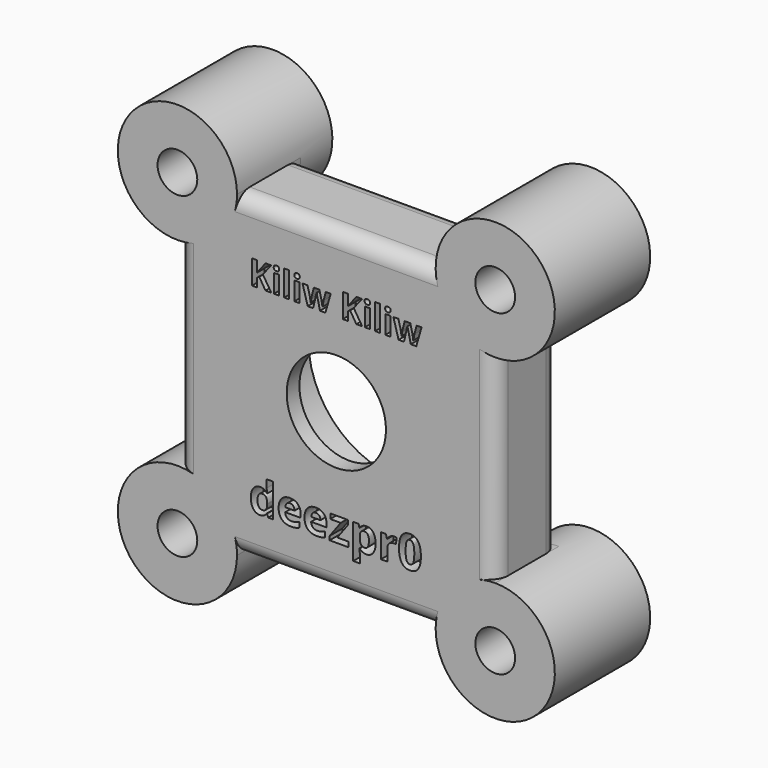
from build123d import *

# Parameters (mm, degrees)
F0_W            = 40
F0_H            = 40
F1_DEPTH        = 5
F2_R            = 11.5
F3_DEPTH        = 8
F4_R            = 6.25
F5_DEPTH        = 25
F7_DEPTH        = 15
F8_R            = 2.5
F9_DEPTH        = 35
F10_T4_DEPTH    = 35
F10_S5_R        = 7.5
F10_T6_DEPTH    = 19
F10_S7_R        = 7.5
F10_T8_DEPTH    = 19
F10_T12_DEPTH   = 35
F10_S13_R       = 7.5
F10_T14_DEPTH   = 19
F10_S15_R       = 7.5
F10_T16_DEPTH   = 19
F10_T20_DEPTH   = 35
F10_S21_R       = 7.5
F10_T22_DEPTH   = 19
F10_S23_R       = 7.5
F10_T24_DEPTH   = 19
F10_T28_DEPTH   = 35
F10_S29_R       = 7.5
F10_T30_DEPTH   = 19
F10_S31_R       = 7.5
F10_T32_DEPTH   = 19
F10_T36_DEPTH   = 35
F10_S37_R       = 7.5
F10_T38_DEPTH   = 19
F10_S39_R       = 7.5
F10_T40_DEPTH   = 19
F10_T44_DEPTH   = 35
F10_S45_R       = 7.5
F10_T46_DEPTH   = 19
F10_S47_R       = 7.5
F10_T48_DEPTH   = 19
F10_T52_DEPTH   = 35
F10_S53_R       = 7.5
F10_T54_DEPTH   = 19
F10_S55_R       = 7.5
F10_T56_DEPTH   = 19
F10_T60_DEPTH   = 35
F10_S61_R       = 7.5
F10_T62_DEPTH   = 19
F10_S63_R       = 7.5
F10_T64_DEPTH   = 19
F11_TEXT_SIZE   = 5.5150802977
F11_TEXT_SIZE_2 = 4.242241639
F12_DEPTH       = 2


# Not quite as in the source:
# - a fillet or chamfer that OpenCascade refuses, or shapes differently, is made with other operations: its cross-section is extruded or revolved along the edge and cut away or added
# - Text() gives the source's letters only with a copy of the font that has no kerning and outlines rounded to 1/6400 em; it was checked with that copy


with BuildPart() as f1:
    # F0 (on Front) → F1 (new body, symmetric)
    with BuildSketch(Plane.XZ):
        Rectangle(F0_W, F0_H)
    extrude(amount=F1_DEPTH, both=True)

    # F2 (on face) → F3 (cut)
    with BuildSketch(Plane(origin=(0, 5, 0), x_dir=(-1, 0, 0), z_dir=(0, 1, 0))):
        Circle(F2_R)
    extrude(amount=-F3_DEPTH, mode=Mode.SUBTRACT)

    # F4 (on face) → F5 (cut)
    with BuildSketch(Plane.XZ.offset(5)):
        Circle(F4_R)
    extrude(amount=-F5_DEPTH, mode=Mode.SUBTRACT)

    # F6 (on face) → F7 (join)
    with BuildSketch(Plane.XZ.offset(5)):
        with BuildLine():
            Line((-20, 20), (-12.5, 20))
            ThreePointArc((-12.5, 20), (-25.3033008589, 25.3033008589), (-20, 12.5))
            Line((-20, 12.5), (-20, 20))
        make_face()
        with BuildLine():
            ThreePointArc((-20, 12.5), (-14.6966991411, 14.6966991411), (-12.5, 20))
            Line((-12.5, 20), (-20, 20))
            Line((-20, 20), (-20, 12.5))
        make_face()
        with BuildLine():
            Line((20, 20), (12.5, 20))
            ThreePointArc((12.5, 20), (14.6966991411, 14.6966991411), (20, 12.5))
            Line((20, 12.5), (20, 20))
        make_face()
        with BuildLine():
            ThreePointArc((27.5, 20), (20, 27.5), (12.5, 20))
            Line((12.5, 20), (20, 20))
            Line((20, 20), (20, 12.5))
            ThreePointArc((20, 12.5), (25.3033008589, 14.6966991411), (27.5, 20))
        make_face()
        with BuildLine():
            ThreePointArc((-12.5, -20), (-14.6966991411, -14.6966991411), (-20, -12.5))
            Line((-20, -12.5), (-20, -20))
            Line((-20, -20), (-12.5, -20))
        make_face()
        with BuildLine():
            Line((-20, -20), (-20, -12.5))
            ThreePointArc((-20, -12.5), (-25.3033008589, -25.3033008589), (-12.5, -20))
            Line((-12.5, -20), (-20, -20))
        make_face()
        with BuildLine():
            Line((20, -20), (20, -12.5))
            ThreePointArc((20, -12.5), (14.6966991411, -14.6966991411), (12.5, -20))
            Line((12.5, -20), (20, -20))
        make_face()
        with BuildLine():
            ThreePointArc((27.5, -20), (25.3033008589, -14.6966991411), (20, -12.5))
            Line((20, -12.5), (20, -20))
            Line((20, -20), (12.5, -20))
            ThreePointArc((12.5, -20), (20, -27.5), (27.5, -20))
        make_face()
    extrude(amount=-F7_DEPTH)

    # F8 (on face) → F9 (cut)
    with BuildSketch(Plane.XZ.offset(5)):
        with Locations((-20, 20)):
            Circle(F8_R)
        with Locations((20, 20)):
            Circle(F8_R)
        with Locations((-20, -20)):
            Circle(F8_R)
        with Locations((20, -20)):
            Circle(F8_R)
    extrude(amount=-F9_DEPTH, mode=Mode.SUBTRACT)

    # F10: fillet of radius 2 on 8 edges, made by hand


with BuildPart() as f10_tool2:
    # F10_s3 → F10_t4 (new body)
    with BuildSketch(Plane.YZ.offset(17.5)):
        with BuildLine():
            ThreePointArc((-5, 18), (-4.4142135624, 19.4142135624), (-3, 20))
            Line((-3, 20), (-5, 20))
            Line((-5, 20), (-5, 18))
        make_face()
    extrude(amount=-F10_T4_DEPTH)

    # F10_s5 → F10_t6 (cut, symmetric)
    with BuildSketch(Plane.XZ.offset(4)):
        with Locations((20, 20)):
            Circle(F10_S5_R)
    extrude(amount=F10_T6_DEPTH, both=True, mode=Mode.SUBTRACT)

    # F10_s7 → F10_t8 (cut, symmetric)
    with BuildSketch(Plane.XZ.offset(4)):
        with Locations((-20, 20)):
            Circle(F10_S7_R)
    extrude(amount=F10_T8_DEPTH, both=True, mode=Mode.SUBTRACT)


with BuildPart() as f1_1:
    add(f1.part)

    # F10_t1: cut F10_tool2
    add(f10_tool2.part, mode=Mode.SUBTRACT)


with BuildPart() as f10_tool10:
    # F10_s11 → F10_t12 (new body)
    with BuildSketch(Plane.YZ.offset(-17.5)):
        with BuildLine():
            ThreePointArc((-5, -18), (-4.4142135624, -19.4142135624), (-3, -20))
            Line((-3, -20), (-5, -20))
            Line((-5, -20), (-5, -18))
        make_face()
    extrude(amount=F10_T12_DEPTH)

    # F10_s13 → F10_t14 (cut, symmetric)
    with BuildSketch(Plane.XZ.offset(4)):
        with Locations((20, -20)):
            Circle(F10_S13_R)
    extrude(amount=F10_T14_DEPTH, both=True, mode=Mode.SUBTRACT)

    # F10_s15 → F10_t16 (cut, symmetric)
    with BuildSketch(Plane.XZ.offset(4)):
        with Locations((-20, -20)):
            Circle(F10_S15_R)
    extrude(amount=F10_T16_DEPTH, both=True, mode=Mode.SUBTRACT)


with BuildPart() as f1_2:
    add(f1_1.part)

    # F10_t9: cut F10_tool10
    add(f10_tool10.part, mode=Mode.SUBTRACT)


with BuildPart() as f10_tool18:
    # F10_s19 → F10_t20 (new body)
    with BuildSketch(Plane.XY.offset(17.5)):
        with BuildLine():
            ThreePointArc((-18, -5), (-19.4142135624, -4.4142135624), (-20, -3))
            Line((-20, -3), (-20, -5))
            Line((-20, -5), (-18, -5))
        make_face()
    extrude(amount=-F10_T20_DEPTH)

    # F10_s21 → F10_t22 (cut, symmetric)
    with BuildSketch(Plane.XZ.offset(4)):
        with Locations((-20, -20)):
            Circle(F10_S21_R)
    extrude(amount=F10_T22_DEPTH, both=True, mode=Mode.SUBTRACT)

    # F10_s23 → F10_t24 (cut, symmetric)
    with BuildSketch(Plane.XZ.offset(4)):
        with Locations((-20, 20)):
            Circle(F10_S23_R)
    extrude(amount=F10_T24_DEPTH, both=True, mode=Mode.SUBTRACT)


with BuildPart() as f1_3:
    add(f1_2.part)

    # F10_t17: cut F10_tool18
    add(f10_tool18.part, mode=Mode.SUBTRACT)


with BuildPart() as f10_tool26:
    # F10_s27 → F10_t28 (new body)
    with BuildSketch(Plane.XY.offset(-17.5)):
        with BuildLine():
            ThreePointArc((18, -5), (19.4142135624, -4.4142135624), (20, -3))
            Line((20, -3), (20, -5))
            Line((20, -5), (18, -5))
        make_face()
    extrude(amount=F10_T28_DEPTH)

    # F10_s29 → F10_t30 (cut, symmetric)
    with BuildSketch(Plane.XZ.offset(4)):
        with Locations((20, -20)):
            Circle(F10_S29_R)
    extrude(amount=F10_T30_DEPTH, both=True, mode=Mode.SUBTRACT)

    # F10_s31 → F10_t32 (cut, symmetric)
    with BuildSketch(Plane.XZ.offset(4)):
        with Locations((20, 20)):
            Circle(F10_S31_R)
    extrude(amount=F10_T32_DEPTH, both=True, mode=Mode.SUBTRACT)


with BuildPart() as f1_4:
    add(f1_3.part)

    # F10_t25: cut F10_tool26
    add(f10_tool26.part, mode=Mode.SUBTRACT)


with BuildPart() as f10_tool34:
    # F10_s35 → F10_t36 (new body)
    with BuildSketch(Plane.XY.offset(-17.5)):
        with BuildLine():
            ThreePointArc((20, 3), (19.4142135624, 4.4142135624), (18, 5))
            Line((18, 5), (20, 5))
            Line((20, 5), (20, 3))
        make_face()
    extrude(amount=F10_T36_DEPTH)

    # F10_s37 → F10_t38 (cut, symmetric)
    with BuildSketch(Plane.XZ.offset(-4)):
        with Locations((20, -20)):
            Circle(F10_S37_R)
    extrude(amount=F10_T38_DEPTH, both=True, mode=Mode.SUBTRACT)

    # F10_s39 → F10_t40 (cut, symmetric)
    with BuildSketch(Plane.XZ.offset(-4)):
        with Locations((20, 20)):
            Circle(F10_S39_R)
    extrude(amount=F10_T40_DEPTH, both=True, mode=Mode.SUBTRACT)


with BuildPart() as f1_5:
    add(f1_4.part)

    # F10_t33: cut F10_tool34
    add(f10_tool34.part, mode=Mode.SUBTRACT)


with BuildPart() as f10_tool42:
    # F10_s43 → F10_t44 (new body)
    with BuildSketch(Plane.XY.offset(17.5)):
        with BuildLine():
            ThreePointArc((-20, 3), (-19.4142135624, 4.4142135624), (-18, 5))
            Line((-18, 5), (-20, 5))
            Line((-20, 5), (-20, 3))
        make_face()
    extrude(amount=-F10_T44_DEPTH)

    # F10_s45 → F10_t46 (cut, symmetric)
    with BuildSketch(Plane.XZ.offset(-4)):
        with Locations((-20, -20)):
            Circle(F10_S45_R)
    extrude(amount=F10_T46_DEPTH, both=True, mode=Mode.SUBTRACT)

    # F10_s47 → F10_t48 (cut, symmetric)
    with BuildSketch(Plane.XZ.offset(-4)):
        with Locations((-20, 20)):
            Circle(F10_S47_R)
    extrude(amount=F10_T48_DEPTH, both=True, mode=Mode.SUBTRACT)


with BuildPart() as f1_6:
    add(f1_5.part)

    # F10_t41: cut F10_tool42
    add(f10_tool42.part, mode=Mode.SUBTRACT)


with BuildPart() as f10_tool50:
    # F10_s51 → F10_t52 (new body)
    with BuildSketch(Plane.YZ.offset(17.5)):
        with BuildLine():
            ThreePointArc((3, 20), (4.4142135624, 19.4142135624), (5, 18))
            Line((5, 18), (5, 20))
            Line((5, 20), (3, 20))
        make_face()
    extrude(amount=-F10_T52_DEPTH)

    # F10_s53 → F10_t54 (cut, symmetric)
    with BuildSketch(Plane.XZ.offset(-4)):
        with Locations((20, 20)):
            Circle(F10_S53_R)
    extrude(amount=F10_T54_DEPTH, both=True, mode=Mode.SUBTRACT)

    # F10_s55 → F10_t56 (cut, symmetric)
    with BuildSketch(Plane.XZ.offset(-4)):
        with Locations((-20, 20)):
            Circle(F10_S55_R)
    extrude(amount=F10_T56_DEPTH, both=True, mode=Mode.SUBTRACT)


with BuildPart() as f1_7:
    add(f1_6.part)

    # F10_t49: cut F10_tool50
    add(f10_tool50.part, mode=Mode.SUBTRACT)


with BuildPart() as f10_tool58:
    # F10_s59 → F10_t60 (new body)
    with BuildSketch(Plane.YZ.offset(-17.5)):
        with BuildLine():
            ThreePointArc((3, -20), (4.4142135624, -19.4142135624), (5, -18))
            Line((5, -18), (5, -20))
            Line((5, -20), (3, -20))
        make_face()
    extrude(amount=F10_T60_DEPTH)

    # F10_s61 → F10_t62 (cut, symmetric)
    with BuildSketch(Plane.XZ.offset(-4)):
        with Locations((20, -20)):
            Circle(F10_S61_R)
    extrude(amount=F10_T62_DEPTH, both=True, mode=Mode.SUBTRACT)

    # F10_s63 → F10_t64 (cut, symmetric)
    with BuildSketch(Plane.XZ.offset(-4)):
        with Locations((-20, -20)):
            Circle(F10_S63_R)
    extrude(amount=F10_T64_DEPTH, both=True, mode=Mode.SUBTRACT)


with BuildPart() as f1_8:
    add(f1_7.part)

    # F10_t57: cut F10_tool58
    add(f10_tool58.part, mode=Mode.SUBTRACT)

    # F11 (on face) → F12 (cut)
    with BuildSketch(Plane.XZ.offset(5)):
        with Locations((-11, -14.5420908112)):
            Text('deezpr0', F11_TEXT_SIZE, font='Open Sans', font_style=FontStyle.BOLD, text_align=(TextAlign.LEFT, TextAlign.BOTTOM))
        with Locations((-11, 10.4986885206)):
            Text('Kiliw Kiliw', F11_TEXT_SIZE_2, font='Open Sans', font_style=FontStyle.BOLD, text_align=(TextAlign.LEFT, TextAlign.BOTTOM))
    extrude(amount=-F12_DEPTH, mode=Mode.SUBTRACT)


solid = f1_8.part
